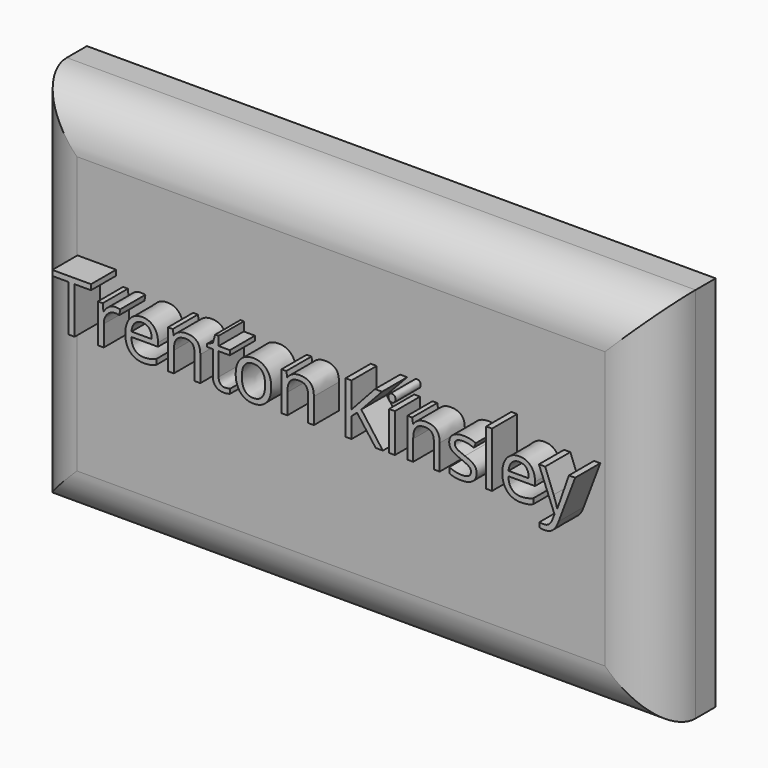
from build123d import *

# Parameters (mm, degrees)
F0_W         = 63.5
F0_H         = 38.1
F1_DEPTH     = 7.62
F2_R         = 5.08
F3_TEXT_SIZE = 7.3004426766
F4_DEPTH     = 3.175


# Not quite as in the source:
# - Text() gives the source's letters only with a copy of the font that has no kerning and outlines rounded to 1/6400 em; it was checked with that copy


with BuildPart() as f1:
    # F0 (on Front) → F1 (new body)
    with BuildSketch(Plane.XZ):
        with Locations((31.75, 19.05)):
            Rectangle(F0_W, F0_H)
    extrude(amount=F1_DEPTH)

    # F2
    f2_edges = [f1.edges().sort_by_distance(p)[0] for p in [
        (0, -7.62, 19.05),
        (31.75, -7.62, 0),
        (63.5, -7.62, 19.05),
        (31.75, -7.62, 38.1),
    ]]
    fillet(f2_edges, radius=F2_R)

    # F3 (on face) → F4 (join)
    with BuildSketch(Plane.XZ.offset(7.62)):
        with Locations((5.08, 19.05)):
            Text('Trenton Kinsley', F3_TEXT_SIZE, font='Open Sans', text_align=(TextAlign.LEFT, TextAlign.BOTTOM))
    extrude(amount=F4_DEPTH)


solid = f1.part
